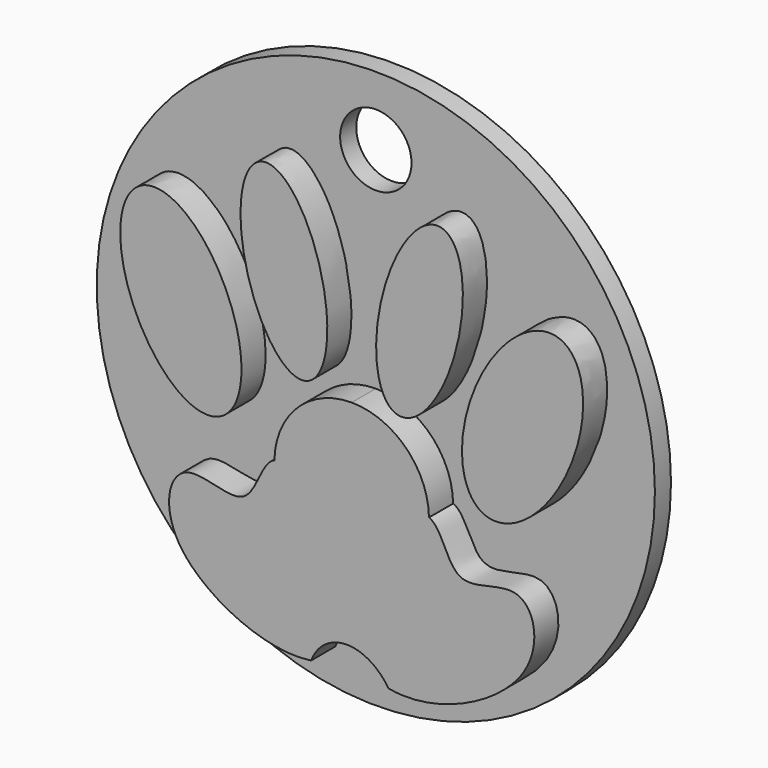
from build123d import *

# Parameters (mm, degrees)
F1_DEPTH = 6.35
F2_R     = 40.9832511975
F2_R_2   = 35.5935039739
F3_DEPTH = 6.35
F5_R     = 35.2656682334
F6_DEPTH = 2.54
F7_R     = 4.5069254771
F8_DEPTH = 2.54


with BuildPart() as f1:
    # F0 (on Front) → F1 (new body)
    with BuildSketch(Plane.XZ):
        with BuildLine():
            add(Edge.make_bspline(
                [(0, 0), (-0.8542329599, -0.0309298364), (-1.2996616548, -4.4613797175), (-2.3936062671, -7.4517694667)],
                knots=[0.7613049359, 0.7613049359, 0.7613049359, 0.7613049359, 0.8627917453, 0.8627917453, 0.8627917453, 0.8627917453], degree=3))
            ThreePointArc((0, 0), (-0.0092947165, -4.4224e-06), (-0.0185894245, -1.76894e-05))
            add(Edge.make_bspline(
                [(-2.3936062671, -7.4517694667), (-1.7627806242, -3.1928435627), (-0.7469629996, -0.0275428514), (-0.0185894245, -1.76894e-05)],
                knots=[0.6746259926, 0.6746259926, 0.6746259926, 0.6746259926, 0.7605712877, 0.7605712877, 0.7605712877, 0.7605712877], degree=3))
        make_face()
        with BuildLine():
            Line((0, -27.1692338988), (0, 0))
            add(Edge.make_bspline(
                [(0, 0), (-0.8542329599, -0.0309298364), (-1.2996616548, -4.4613797175), (-2.3936062671, -7.4517694667)],
                knots=[0.7613049359, 0.7613049359, 0.7613049359, 0.7613049359, 0.8627917453, 0.8627917453, 0.8627917453, 0.8627917453], degree=3))
            add(Edge.make_bspline(
                [(-0.3373747703, -27.1383245315), (-3.4203099334, -22.7407711946), (-3.342600692, -13.8587647826), (-2.3936062671, -7.4517694667)],
                knots=[0.5453325708, 0.5453325708, 0.5453325708, 0.5453325708, 0.6746259926, 0.6746259926, 0.6746259926, 0.6746259926], degree=3))
            add(Edge.make_bspline(
                [(-0.337374764, -27.1383245227), (-0.225223024, -27.1449008745), (-0.1127129786, -27.1552026154), (0, -27.1692338988)],
                knots=[0.1251291941, 0.1251291941, 0.1251291941, 0.1251291941, 0.1320936712, 0.1320936712, 0.1320936712, 0.1320936712], degree=3))
        make_face()
        with BuildLine():
            add(Edge.make_bspline(
                [(0, 0), (0.8542329599, -0.0309298364), (1.2996616548, -4.4613797175), (2.3936062671, -7.4517694667)],
                knots=[0.7613049359, 0.7613049359, 0.7613049359, 0.7613049359, 0.8627917453, 0.8627917453, 0.8627917453, 0.8627917453], degree=3))
            Line((0, 0), (0, -27.1692338988))
            add(Edge.make_bspline(
                [(0, -27.1692338988), (0.0947968893, -27.1810348647), (0.1897373254, -27.1954739587), (0.2847288735, -27.2125536519)],
                knots=[0.1320936712, 0.1320936712, 0.1320936712, 0.1320936712, 0.1379511223, 0.1379511223, 0.1379511223, 0.1379511223], degree=3))
            add(Edge.make_bspline(
                [(0.284728874, -27.2125536558), (3.4211615885, -22.8413824024), (3.3479713394, -13.8950239132), (2.3936062671, -7.4517694667)],
                knots=[0.5446008601, 0.5446008601, 0.5446008601, 0.5446008601, 0.6746259926, 0.6746259926, 0.6746259926, 0.6746259926], degree=3))
        make_face()
        with BuildLine():
            ThreePointArc((0.0185894245, -1.76894e-05), (0.0092947165, -4.4224e-06), (0, 0))
            add(Edge.make_bspline(
                [(0, 0), (0.8542329599, -0.0309298364), (1.2996616548, -4.4613797175), (2.3936062671, -7.4517694667)],
                knots=[0.7613049359, 0.7613049359, 0.7613049359, 0.7613049359, 0.8627917453, 0.8627917453, 0.8627917453, 0.8627917453], degree=3))
            add(Edge.make_bspline(
                [(2.3936062671, -7.4517694667), (1.7627806242, -3.1928435627), (0.7469629996, -0.0275428514), (0.0185894245, -1.76894e-05)],
                knots=[0.6746259926, 0.6746259926, 0.6746259926, 0.6746259926, 0.7605712877, 0.7605712877, 0.7605712877, 0.7605712877], degree=3))
        make_face()
        with BuildLine():
            add(Edge.make_bspline(
                [(0.2847288735, -27.2125536519), (1.8691527538, -27.497436615), (3.467796537, -28.5169608167), (4.6517230542, -30.2825928689)],
                knots=[0.1379511223, 0.1379511223, 0.1379511223, 0.1379511223, 0.2356512402, 0.2356512402, 0.2356512402, 0.2356512402], degree=3))
            add(Edge.make_bspline(
                [(9.7663515031, -9.6101000815), (11.4558651985, -10.2661306715), (12.43631527, -17.8432939914), (22.3742050925, -11.6036791249), (25.1401756668, -24.4664864351), (10.5320133814, -31.4621716212), (4.6517230542, -30.2825928689)],
                knots=[0, 0, 0, 0, 0.1078809829, 0.2205738258, 0.3436583505, 0.4939703317, 0.4939703317, 0.4939703317, 0.4939703317], degree=3))
            add(Edge.make_bspline(
                [(2.3936062671, -7.4517694667), (2.7640750419, -8.4644770701), (4.5399930942, -11.8480905406), (8.1557945616, -8.9847280448), (9.7663515031, -9.6101000815)],
                knots=[0.8627917453, 0.8627917453, 0.8627917453, 0.8627917453, 0.8971606644, 1, 1, 1, 1], degree=3))
            add(Edge.make_bspline(
                [(0.284728874, -27.2125536558), (3.4211615885, -22.8413824024), (3.3479713394, -13.8950239132), (2.3936062671, -7.4517694667)],
                knots=[0.5446008601, 0.5446008601, 0.5446008601, 0.5446008601, 0.6746259926, 0.6746259926, 0.6746259926, 0.6746259926], degree=3))
        make_face()
        with BuildLine():
            add(Edge.make_bspline(
                [(-9.7663515031, -9.6101000815), (-11.4558651985, -10.2661306715), (-12.43631527, -17.8432939914), (-22.3742050925, -11.6036791249), (-25.1109997325, -24.3308073267), (-10.9635461115, -31.2532862178), (-5.1342780276, -30.3674903339)],
                knots=[0, 0, 0, 0, 0.1078809829, 0.2205738258, 0.3436583505, 0.4898977947, 0.4898977947, 0.4898977947, 0.4898977947], degree=3))
            add(Edge.make_bspline(
                [(-5.1342780276, -30.3674903339), (-4.2517221479, -28.1045870874), (-2.3523798625, -27.0201686872), (-0.337374764, -27.1383245227)],
                knots=[0, 0, 0, 0, 0.1251291941, 0.1251291941, 0.1251291941, 0.1251291941], degree=3))
            add(Edge.make_bspline(
                [(-0.3373747703, -27.1383245315), (-3.4203099334, -22.7407711946), (-3.342600692, -13.8587647826), (-2.3936062671, -7.4517694667)],
                knots=[0.5453325708, 0.5453325708, 0.5453325708, 0.5453325708, 0.6746259926, 0.6746259926, 0.6746259926, 0.6746259926], degree=3))
            add(Edge.make_bspline(
                [(-2.3936062671, -7.4517694667), (-2.7640750419, -8.4644770701), (-4.5399930942, -11.8480905406), (-8.1557945616, -8.9847280448), (-9.7663515031, -9.6101000815)],
                knots=[0.8627917453, 0.8627917453, 0.8627917453, 0.8627917453, 0.8971606644, 1, 1, 1, 1], degree=3))
        make_face()
        with BuildLine():
            add(Edge.make_bspline(
                [(-2.3936062671, -7.4517694667), (-1.7627806242, -3.1928435627), (-0.7469629996, -0.0275428514), (-0.0185894245, -1.76894e-05)],
                knots=[0.6746259926, 0.6746259926, 0.6746259926, 0.6746259926, 0.7605712877, 0.7605712877, 0.7605712877, 0.7605712877], degree=3))
            ThreePointArc((-0.0185894245, -1.76894e-05), (-6.8574549313, -2.811922896), (-9.7663515031, -9.6101000815))
            add(Edge.make_bspline(
                [(-2.3936062671, -7.4517694667), (-2.7640750419, -8.4644770701), (-4.5399930942, -11.8480905406), (-8.1557945616, -8.9847280448), (-9.7663515031, -9.6101000815)],
                knots=[0.8627917453, 0.8627917453, 0.8627917453, 0.8627917453, 0.8971606644, 1, 1, 1, 1], degree=3))
        make_face()
        with BuildLine():
            ThreePointArc((9.7663515031, -9.6101000815), (6.8574549313, -2.811922896), (0.0185894245, -1.76894e-05))
            add(Edge.make_bspline(
                [(2.3936062671, -7.4517694667), (1.7627806242, -3.1928435627), (0.7469629996, -0.0275428514), (0.0185894245, -1.76894e-05)],
                knots=[0.6746259926, 0.6746259926, 0.6746259926, 0.6746259926, 0.7605712877, 0.7605712877, 0.7605712877, 0.7605712877], degree=3))
            add(Edge.make_bspline(
                [(2.3936062671, -7.4517694667), (2.7640750419, -8.4644770701), (4.5399930942, -11.8480905406), (8.1557945616, -8.9847280448), (9.7663515031, -9.6101000815)],
                knots=[0.8627917453, 0.8627917453, 0.8627917453, 0.8627917453, 0.8971606644, 1, 1, 1, 1], degree=3))
        make_face()
    extrude(amount=F1_DEPTH)


with BuildPart() as f1b:
    # F0 (on Front) → F1, piece 2 (new body)
    with BuildSketch(Plane.XZ):
        with BuildLine():
            add(Edge.make_bspline(
                [(-16.7901068926, -7.026379928), (-6.4540098393, -2.6413687215), (-18.8178188619, 12.1275598328), (-31.1816278845, 26.8964883871), (-29.1539159152, 7.7425486263), (-27.1262039459, -11.4113911344), (-16.7901068926, -7.026379928)],
                knots=[0, 0, 0, 2.0943951024, 2.0943951024, 4.1887902048, 4.1887902048, 6.2831853072, 6.2831853072, 6.2831853072], degree=2, weights=[1, 0.5, 1, 0.5, 1, 0.5, 1]))
        make_face()
    extrude(amount=F1_DEPTH)


with BuildPart() as f1c:
    # F0 (on Front) → F1, piece 3 (new body)
    with BuildSketch(Plane.XZ):
        with BuildLine():
            add(Edge.make_bspline(
                [(-5.8251381852, 0.5120352725), (2.3996030872, 2.5059121089), (-5.8246309889, 18.4704089833), (-14.048865065, 34.4349058578), (-14.0493722613, 16.476532147), (-14.0498794576, -1.4818415638), (-5.8251381852, 0.5120352725)],
                knots=[0, 0, 0, 2.0943951024, 2.0943951024, 4.1887902048, 4.1887902048, 6.2831853072, 6.2831853072, 6.2831853072], degree=2, weights=[1, 0.5, 1, 0.5, 1, 0.5, 1]))
        make_face()
    extrude(amount=F1_DEPTH)


with BuildPart() as f1d:
    # F0 (on Front) → F1, piece 4 (new body)
    with BuildSketch(Plane.XZ):
        with BuildLine():
            add(Edge.make_bspline(
                [(5.8251381852, 0.5120352725), (14.0498794576, -1.4818415638), (14.0493722613, 16.476532147), (14.048865065, 34.4349058578), (5.8246309889, 18.4704089833), (-2.3996030872, 2.5059121089), (5.8251381852, 0.5120352725)],
                knots=[0, 0, 0, 2.0943951024, 2.0943951024, 4.1887902048, 4.1887902048, 6.2831853072, 6.2831853072, 6.2831853072], degree=2, weights=[1, 0.5, 1, 0.5, 1, 0.5, 1]))
        make_face()
    extrude(amount=F1_DEPTH)


with BuildPart() as f1e:
    # F0 (on Front) → F1, piece 5 (new body)
    with BuildSketch(Plane.XZ):
        with BuildLine():
            add(Edge.make_bspline(
                [(16.7901068926, -7.026379928), (27.1262039459, -11.4113911344), (29.1539159152, 7.7425486263), (31.1816278845, 26.8964883871), (18.8178188619, 12.1275598328), (6.4540098393, -2.6413687215), (16.7901068926, -7.026379928)],
                knots=[0, 0, 0, 2.0943951024, 2.0943951024, 4.1887902048, 4.1887902048, 6.2831853072, 6.2831853072, 6.2831853072], degree=2, weights=[1, 0.5, 1, 0.5, 1, 0.5, 1]))
        make_face()
    extrude(amount=F1_DEPTH)


with BuildPart() as f3:
    # F2 (on Front) → F3 (new body)
    with BuildSketch(Plane.XZ):
        Circle(F2_R)
        Circle(F2_R_2, mode=Mode.SUBTRACT)
    extrude(amount=F3_DEPTH)


with BuildPart() as f6:
    # F5 (on Front) → F6 (new body)
    with BuildSketch(Plane.XZ):
        Circle(F5_R)
    extrude(amount=F6_DEPTH)

    # F7 (on Front) → F8 (cut)
    with BuildSketch(Plane.XZ):
        with Locations((0, 26.5538338572)):
            Circle(F7_R)
    extrude(amount=F8_DEPTH, mode=Mode.SUBTRACT)


solid = Compound([f1.part, f1b.part, f1c.part, f1d.part, f1e.part, f6.part])
